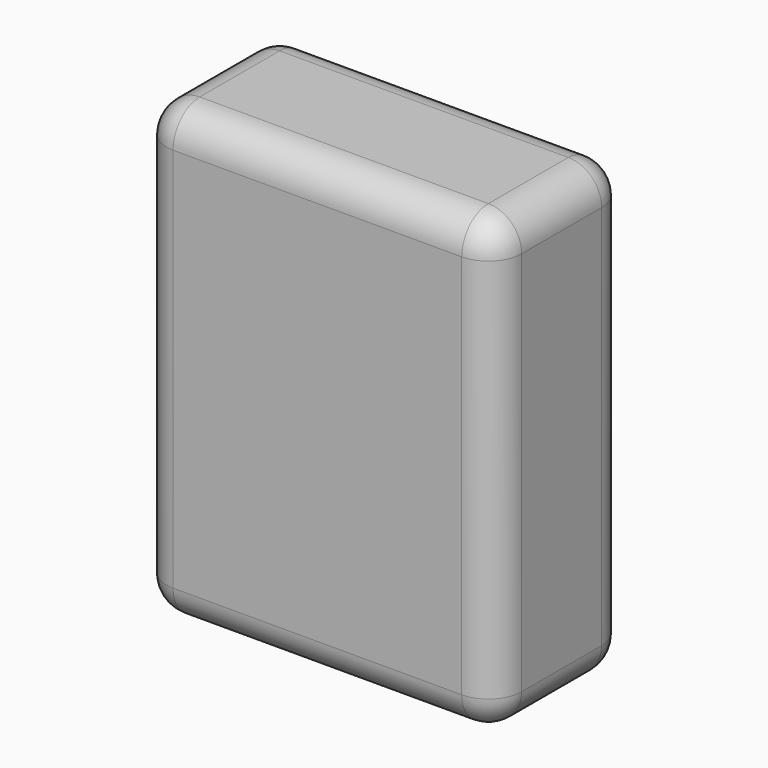
from build123d import *

# Parameters (mm, degrees)
F0_W         = 54.1939660907
F0_H         = 68.9741391689
F1_DEPTH     = 25.4
F2_R         = 5.08
F3_T1_DEPTH  = 58.8141391689
F3_T3_DEPTH  = 44.0339660907
F3_T5_DEPTH  = 15.24
F3_S9_W      = 5.08
F3_S9_H      = 5.08
F3_T10_DEPTH = 5.08
F3_S15_W     = 5.08
F3_S15_H     = 5.08
F3_T16_DEPTH = 5.08
F3_S21_W     = 5.08
F3_S21_H     = 5.08
F3_T22_DEPTH = 5.08
F3_S27_W     = 5.08
F3_S27_H     = 5.08
F3_T28_DEPTH = 5.08
F3_S33_W     = 5.08
F3_S33_H     = 5.08
F3_T34_DEPTH = 5.08
F3_S39_W     = 5.08
F3_S39_H     = 5.08
F3_T40_DEPTH = 5.08
F3_T44_ANGLE = 90
F3_T46_ANGLE = 90


# Not quite as in the source:
# - a fillet or chamfer that OpenCascade refuses, or shapes differently, is made with other operations: its cross-section is extruded or revolved along the edge and cut away or added


with BuildPart() as f1:
    # F0 (on Front) → F1 (new body)
    with BuildSketch(Plane.XZ):
        with Locations((-4.6311207116, -5.9120682999)):
            Rectangle(F0_W, F0_H)
    extrude(amount=F1_DEPTH)

    # F2
    f2_edges = [f1.edges().sort_by_distance(p)[0] for p in [
        (22.465862, -12.7, 28.575001),
        (22.465862, 0, -5.912068),
        (-4.631121, -25.4, 28.575001),
    ]]
    fillet(f2_edges, radius=F2_R)

    # F3: fillet of radius 5.08 on 8 edges, made by hand

    # F3_s2 → F3_t1 (cut)
    with BuildSketch(Plane.XY.offset(-35.3191378844)):
        with BuildLine():
            ThreePointArc((17.3858623338, -25.4), (20.9779647822, -23.9121024484), (22.4658623338, -20.32))
            Line((22.4658623338, -20.32), (22.4658623338, -25.4))
            Line((22.4658623338, -25.4), (17.3858623338, -25.4))
        make_face()
        with BuildLine():
            ThreePointArc((-31.7281037569, -5.08), (-30.2402062053, -1.4878975516), (-26.6481037569, 0))
            Line((-26.6481037569, 0), (-31.7281037569, 0))
            Line((-31.7281037569, 0), (-31.7281037569, -5.08))
        make_face()
        with BuildLine():
            ThreePointArc((-31.7281037569, -20.32), (-30.2402062053, -23.9121024484), (-26.6481037569, -25.4))
            Line((-26.6481037569, -25.4), (-31.7281037569, -25.4))
            Line((-31.7281037569, -25.4), (-31.7281037569, -20.32))
        make_face()
    extrude(amount=F3_T1_DEPTH, mode=Mode.SUBTRACT)

    # F3_s4 → F3_t3 (cut)
    with BuildSketch(Plane.YZ.offset(-26.6481037569)):
        with BuildLine():
            ThreePointArc((-5.08, 28.5750012845), (-1.4878975516, 27.0871037329), (0, 23.4950012845))
            Line((0, 23.4950012845), (0, 28.5750012845))
            Line((0, 28.5750012845), (-5.08, 28.5750012845))
        make_face()
        with BuildLine():
            ThreePointArc((-25.4, -35.3191378844), (-23.9121024484, -38.9112403328), (-20.32, -40.3991378844))
            Line((-20.32, -40.3991378844), (-25.4, -40.3991378844))
            Line((-25.4, -40.3991378844), (-25.4, -35.3191378844))
        make_face()
        with BuildLine():
            ThreePointArc((0, -35.3191378844), (-1.4878975516, -38.9112403328), (-5.08, -40.3991378844))
            Line((-5.08, -40.3991378844), (0, -40.3991378844))
            Line((0, -40.3991378844), (0, -35.3191378844))
        make_face()
    extrude(amount=F3_T3_DEPTH, mode=Mode.SUBTRACT)

    # F3_s6 → F3_t5 (cut)
    with BuildSketch(Plane.XZ.offset(5.08)):
        with BuildLine():
            ThreePointArc((-26.6481037569, 28.5750012845), (-30.2402062053, 27.0871037329), (-31.7281037569, 23.4950012845))
            Line((-31.7281037569, 23.4950012845), (-31.7281037569, 28.5750012845))
            Line((-31.7281037569, 28.5750012845), (-26.6481037569, 28.5750012845))
        make_face()
        with BuildLine():
            ThreePointArc((17.3858623338, -40.3991378844), (20.9779647822, -38.9112403328), (22.4658623338, -35.3191378844))
            Line((22.4658623338, -35.3191378844), (22.4658623338, -40.3991378844))
            Line((22.4658623338, -40.3991378844), (17.3858623338, -40.3991378844))
        make_face()
        with BuildLine():
            ThreePointArc((-31.7281037569, -35.3191378844), (-30.2402062053, -38.9112403328), (-26.6481037569, -40.3991378844))
            Line((-26.6481037569, -40.3991378844), (-31.7281037569, -40.3991378844))
            Line((-31.7281037569, -40.3991378844), (-31.7281037569, -35.3191378844))
        make_face()
    extrude(amount=F3_T5_DEPTH, mode=Mode.SUBTRACT)


with BuildPart() as f3_tool8:
    # F3_s9 → F3_t10 (new body)
    with BuildSketch(Plane.XY.offset(23.4950012845)):
        with Locations((19.9258623338, -2.54)):
            Rectangle(F3_S9_W, F3_S9_H)
    extrude(amount=F3_T10_DEPTH)

    # F3_s11 → F3_t12 (revolve, cut)
    with BuildSketch(Plane(origin=(17.3858623338, -5.08, 23.4950012845), x_dir=(-0.7071067812, -0.7071067812, 0), z_dir=(-0.7071067812, 0.7071067812, 0))):
        with BuildLine():
            ThreePointArc((0, -5.08), (5.08, 0), (0, 5.08))
            Line((0, 5.08), (0, -5.08))
        make_face()
    revolve(axis=Axis((17.3858623338, -5.08, 23.4950012845), (0, 0, 1)), mode=Mode.SUBTRACT)


with BuildPart() as f1_1:
    add(f1.part)

    # F3_t7: cut F3_tool8
    add(f3_tool8.part, mode=Mode.SUBTRACT)


with BuildPart() as f3_tool14:
    # F3_s15 → F3_t16 (new body)
    with BuildSketch(Plane.XZ.offset(20.32)):
        with Locations((19.9258623338, 26.0350012845)):
            Rectangle(F3_S15_W, F3_S15_H)
    extrude(amount=F3_T16_DEPTH)

    # F3_s17 → F3_t18 (revolve, cut)
    with BuildSketch(Plane(origin=(17.3858623338, -20.32, 23.4950012845), x_dir=(-0.7071067812, 0, -0.7071067812), z_dir=(-0.7071067812, 0, 0.7071067812))):
        with BuildLine():
            ThreePointArc((0, -5.08), (5.08, 0), (0, 5.08))
            Line((0, 5.08), (0, -5.08))
        make_face()
    revolve(axis=Axis((17.3858623338, -20.32, 23.4950012845), (0, -1, 0)), mode=Mode.SUBTRACT)


with BuildPart() as f1_2:
    add(f1_1.part)

    # F3_t13: cut F3_tool14
    add(f3_tool14.part, mode=Mode.SUBTRACT)


with BuildPart() as f3_tool20:
    # F3_s21 → F3_t22 (new body)
    with BuildSketch(Plane.YZ.offset(17.3858623338)):
        with Locations((-22.86, -37.8591378844)):
            Rectangle(F3_S21_W, F3_S21_H)
    extrude(amount=F3_T22_DEPTH)

    # F3_s23 → F3_t24 (revolve, cut)
    with BuildSketch(Plane(origin=(17.3858623338, -20.32, -35.3191378844), x_dir=(0, 0.7071067812, 0.7071067812), z_dir=(0, 0.7071067812, -0.7071067812))):
        with BuildLine():
            ThreePointArc((0, -5.08), (5.08, 0), (0, 5.08))
            Line((0, 5.08), (0, -5.08))
        make_face()
    revolve(axis=Axis((17.3858623338, -20.32, -35.3191378844), (1, 0, 0)), mode=Mode.SUBTRACT)


with BuildPart() as f1_3:
    add(f1_2.part)

    # F3_t19: cut F3_tool20
    add(f3_tool20.part, mode=Mode.SUBTRACT)


with BuildPart() as f3_tool26:
    # F3_s27 → F3_t28 (new body)
    with BuildSketch(Plane.XY.offset(23.4950012845)):
        with Locations((-29.1881037569, -2.54)):
            Rectangle(F3_S27_W, F3_S27_H)
    extrude(amount=F3_T28_DEPTH)

    # F3_s29 → F3_t30 (revolve, cut)
    with BuildSketch(Plane(origin=(-26.6481037569, -5.08, 23.4950012845), x_dir=(0.7071067812, -0.7071067812, 0), z_dir=(-0.7071067812, -0.7071067812, 0))):
        with BuildLine():
            ThreePointArc((0, -5.08), (5.08, 0), (0, 5.08))
            Line((0, 5.08), (0, -5.08))
        make_face()
    revolve(axis=Axis((-26.6481037569, -5.08, 23.4950012845), (0, 0, 1)), mode=Mode.SUBTRACT)


with BuildPart() as f1_4:
    add(f1_3.part)

    # F3_t25: cut F3_tool26
    add(f3_tool26.part, mode=Mode.SUBTRACT)


with BuildPart() as f3_tool32:
    # F3_s33 → F3_t34 (new body)
    with BuildSketch(Plane.YZ.offset(-26.6481037569)):
        with Locations((-2.54, -37.8591378844)):
            Rectangle(F3_S33_W, F3_S33_H)
    extrude(amount=-F3_T34_DEPTH)

    # F3_s35 → F3_t36 (revolve, cut)
    with BuildSketch(Plane(origin=(-26.6481037569, -5.08, -35.3191378844), x_dir=(0, -0.7071067812, 0.7071067812), z_dir=(0, -0.7071067812, -0.7071067812))):
        with BuildLine():
            ThreePointArc((0, -5.08), (5.08, 0), (0, 5.08))
            Line((0, 5.08), (0, -5.08))
        make_face()
    revolve(axis=Axis((-26.6481037569, -5.08, -35.3191378844), (-1, 0, 0)), mode=Mode.SUBTRACT)


with BuildPart() as f1_5:
    add(f1_4.part)

    # F3_t31: cut F3_tool32
    add(f3_tool32.part, mode=Mode.SUBTRACT)


with BuildPart() as f3_tool38:
    # F3_s39 → F3_t40 (new body)
    with BuildSketch(Plane.YZ.offset(-26.6481037569)):
        with Locations((-22.86, -37.8591378844)):
            Rectangle(F3_S39_W, F3_S39_H)
    extrude(amount=-F3_T40_DEPTH)

    # F3_s41 → F3_t42 (revolve, cut)
    with BuildSketch(Plane(origin=(-26.6481037569, -20.32, -35.3191378844), x_dir=(0, 0.7071067812, 0.7071067812), z_dir=(0, -0.7071067812, 0.7071067812))):
        with BuildLine():
            ThreePointArc((0, -5.08), (5.08, 0), (0, 5.08))
            Line((0, 5.08), (0, -5.08))
        make_face()
    revolve(axis=Axis((-26.6481037569, -20.32, -35.3191378844), (-1, 0, 0)), mode=Mode.SUBTRACT)


with BuildPart() as f1_6:
    add(f1_5.part)

    # F3_t37: cut F3_tool38
    add(f3_tool38.part, mode=Mode.SUBTRACT)

    # F3_s43 → F3_t44 (revolve, cut)
    with BuildSketch(Plane.XZ.offset(5.08)):
        with BuildLine():
            ThreePointArc((17.3858623338, -40.3991378844), (20.9779647822, -38.9112403328), (22.4658623338, -35.3191378844))
            Line((22.4658623338, -35.3191378844), (22.4658623338, -40.3991378844))
            Line((22.4658623338, -40.3991378844), (17.3858623338, -40.3991378844))
        make_face()
    revolve(axis=Axis((17.3858623338, -5.08, -40.3991378844), (0, 0, 1)), revolution_arc=F3_T44_ANGLE, mode=Mode.SUBTRACT)

    # F3_s45 → F3_t46 (revolve, cut)
    with BuildSketch(Plane.XZ.offset(20.32)):
        with BuildLine():
            ThreePointArc((-31.7281037569, 23.4950012845), (-30.2402062053, 27.0871037329), (-26.6481037569, 28.5750012845))
            Line((-26.6481037569, 28.5750012845), (-31.7281037569, 28.5750012845))
            Line((-31.7281037569, 28.5750012845), (-31.7281037569, 23.4950012845))
        make_face()
    revolve(axis=Axis((-31.7281037569, -20.32, 23.4950012845), (1, 0, 0)), revolution_arc=F3_T46_ANGLE, mode=Mode.SUBTRACT)


solid = f1_6.part
